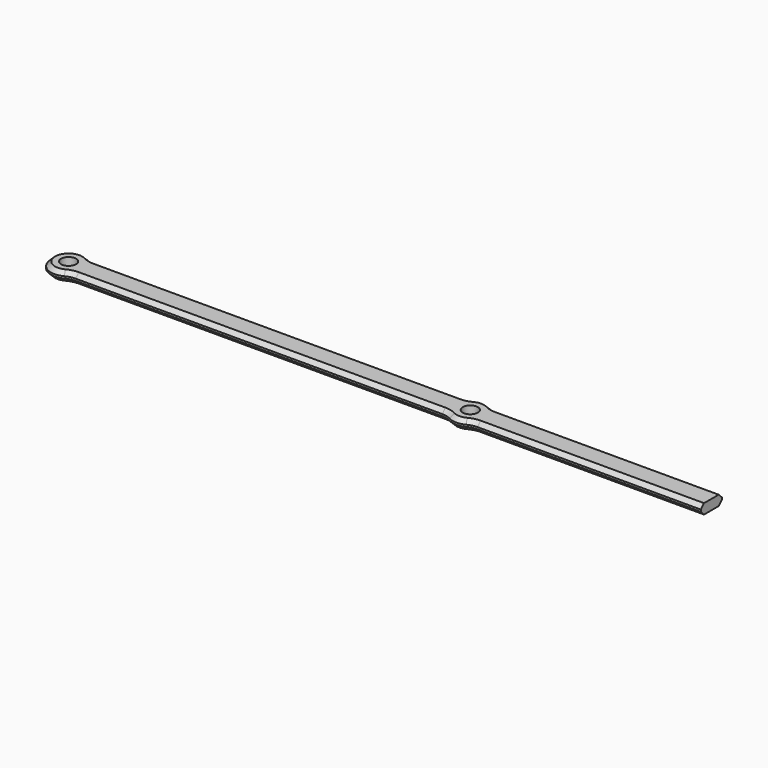
from build123d import *

# Parameters (mm, degrees)
F0_R     = 2.38125
F1_DEPTH = 3.175
F2_R     = 6.35
F3_SIZE  = 1.27


with BuildPart() as f1:
    # F0 (on Top) → F1 (new body)
    with BuildSketch(Plane.XY):
        with BuildLine():
            Line((123.3248860695, 4.1671875), (3.6751139305, 4.1671875))
            ThreePointArc((3.6751139305, 4.1671875), (-5.55625, 0), (3.6751139305, -4.1671875))
            Line((3.6751139305, -4.1671875), (123.3248860695, -4.1671875))
            ThreePointArc((123.3248860695, -4.1671875), (127, -5.55625), (130.6751139305, -4.1671875))
            Line((130.6751139305, -4.1671875), (203.2, -4.1671875))
            Line((203.2, -4.1671875), (203.2, 4.1671875))
            Line((203.2, 4.1671875), (130.6751139305, 4.1671875))
            ThreePointArc((130.6751139305, 4.1671875), (127, 5.55625), (123.3248860695, 4.1671875))
        make_face()
        Circle(F0_R, mode=Mode.SUBTRACT)
        with Locations((127, 0)):
            Circle(F0_R, mode=Mode.SUBTRACT)
    extrude(amount=F1_DEPTH)

    # F2
    f2_edges = [f1.edges().sort_by_distance(p)[0] for p in [
        (3.675114, 4.167187, 1.5875),
        (3.675114, -4.167188, 1.5875),
        (123.324886, -4.167187, 1.5875),
        (130.675114, 4.167187, 1.5875),
        (123.324886, 4.167187, 1.5875),
        (130.675114, -4.167187, 1.5875),
    ]]
    fillet(f2_edges, radius=F2_R)

    # F3
    f3_edges = [f1.edges().sort_by_distance(p)[0] for p in [
        (63.5, 4.167187, 3.175),
        (63.5, 4.167187, 0),
        (127, 5.55625, 0),
        (127, 5.55625, 3.175),
        (131.047329, 4.355179, 0),
        (122.952671, 4.355179, 0),
        (167.8905, 4.167187, 0),
        (4.047329, 4.355179, 0),
        (167.8905, -4.167187, 0),
        (-5.55625, 0, 0),
        (131.047329, -4.355179, 0),
        (4.047329, -4.355179, 0),
        (127, -5.55625, 0),
        (63.5, -4.167187, 0),
        (122.952671, -4.355179, 0),
        (131.047329, 4.355179, 3.175),
        (122.952671, 4.355179, 3.175),
        (167.8905, 4.167187, 3.175),
        (4.047329, 4.355179, 3.175),
        (167.8905, -4.167187, 3.175),
        (-5.55625, 0, 3.175),
        (131.047329, -4.355179, 3.175),
        (4.047329, -4.355179, 3.175),
        (127, -5.55625, 3.175),
        (63.5, -4.167187, 3.175),
        (122.952671, -4.355179, 3.175),
    ]]
    chamfer(f3_edges, length=F3_SIZE)


solid = f1.part
